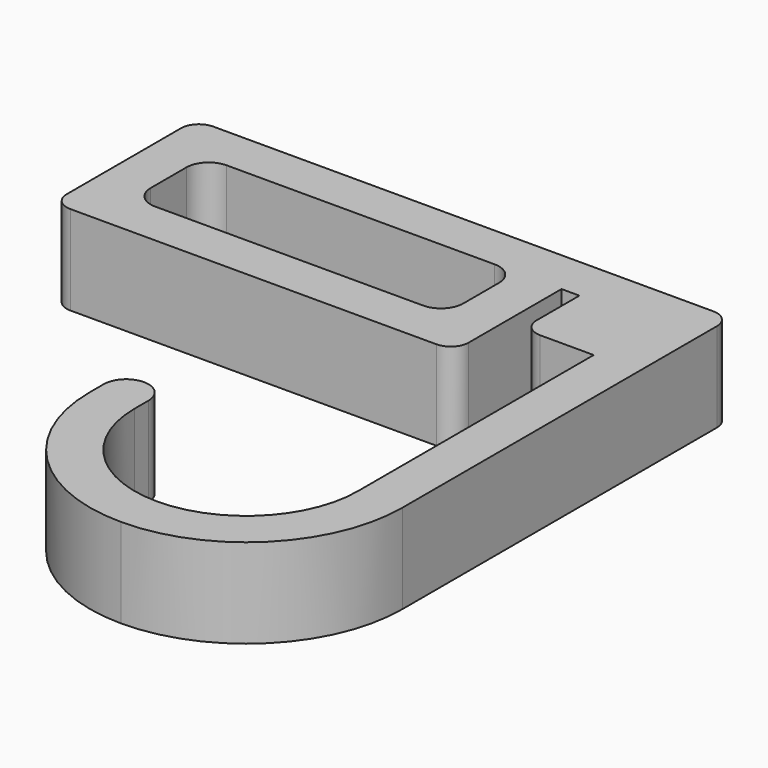
from build123d import *

# Parameters (mm, degrees)
F0_W     = 8
F0_H     = 8
F1_DEPTH = 10
F2_R     = 2
F3_R     = 17.49999
F4_R     = 2.49999


# Not quite as in the source:
# - a fillet or chamfer is up to 0.001 mm smaller than in the source, because OpenCascade refuses the exact size
# - a feature names something its author has since deleted; it is built from what else it names


with BuildPart() as f1:
    # F0 (on Top) → F1 (new body)
    with BuildSketch(Plane.XY):
        Polygon((-18.3916796818, -10.2785023413), (-23.3916796818, -10.2785023413), (-23.3916796818, -25.2785023413), (21.6083203182, -25.2785023413), (21.6083203182, -18.2785023413), (21.6083203182, -10.2785023413), (16.6083203182, -10.2785023413), (16.6083203182, -20.2785023413), (-18.3916796818, -20.2785023413), align=None)
        Polygon((-23.3916796818, -5.2785023413), (-23.3916796818, -10.2785023413), (-18.3916796818, -10.2785023413), (16.6083203182, -10.2785023413), (21.6083203182, -10.2785023413), (23.6083203182, -10.2785023413), (31.6083203182, -10.2785023413), (36.6083203182, -10.2785023413), (36.6083203182, -5.2785023413), align=None)
        with Locations((27.6083203182, -14.2785023413)):
            Rectangle(F0_W, F0_H)
        Polygon((36.6083203182, -36.2785023413), (36.6083203182, -10.2785023413), (31.6083203182, -10.2785023413), (31.6083203182, -18.2785023413), (31.6083203182, -36.2785023413), align=None)
        with BuildLine():
            Line((36.6083203182, -68.7785023413), (36.6083203182, -36.2785023413))
            Line((36.6083203182, -36.2785023413), (31.6083203182, -36.2785023413))
            Line((31.6083203182, -36.2785023413), (31.6083203182, -46.8433834612))
            Line((31.6083203182, -46.8433834612), (31.6083203182, -51.2785023413))
            ThreePointArc((31.6083203182, -51.2785023413), (19.1083203182, -63.7785023413), (6.6083203182, -51.2785023413))
            Line((6.6083203182, -51.2785023413), (6.6083203182, -46.8433834612))
            Line((6.6083203182, -46.8433834612), (1.6083203182, -46.8433834612))
            Line((1.6083203182, -46.8433834612), (1.6083203182, -68.7785023413))
            Line((1.6083203182, -68.7785023413), (36.6083203182, -68.7785023413))
        make_face()
    extrude(amount=F1_DEPTH)

    # F2
    f2_edges = [f1.edges().sort_by_distance(p)[0] for p in [
        (-23.39168, -25.278502, 5),
        (21.60832, -25.278502, 5),
        (23.60832, -18.278502, 5),
        (36.60832, -5.278502, 5),
        (-23.39168, -5.278502, 5),
    ]]
    fillet(f2_edges, radius=F2_R)

    # F3 (radius 17.5 in the source; OpenCascade refuses exactly that, so slightly less here)
    f3_edges = [f1.edges().sort_by_distance(p)[0] for p in [
        (1.60832, -68.778502, 5),
        (36.60832, -68.778502, 5),
    ]]
    fillet(f3_edges, radius=F3_R)

    # F4 (radius 2.5 in the source; OpenCascade refuses exactly that, so slightly less here)
    f4_edges = [f1.edges().sort_by_distance(p)[0] for p in [
        (1.60832, -46.843383, 5),
        (6.60832, -46.843383, 5),
        (-18.39168, -20.278502, 5),
        (-18.39168, -10.278502, 5),
        (16.60832, -10.278502, 5),
        (16.60832, -20.278502, 5),
    ]]
    fillet(f4_edges, radius=F4_R)


solid = f1.part
